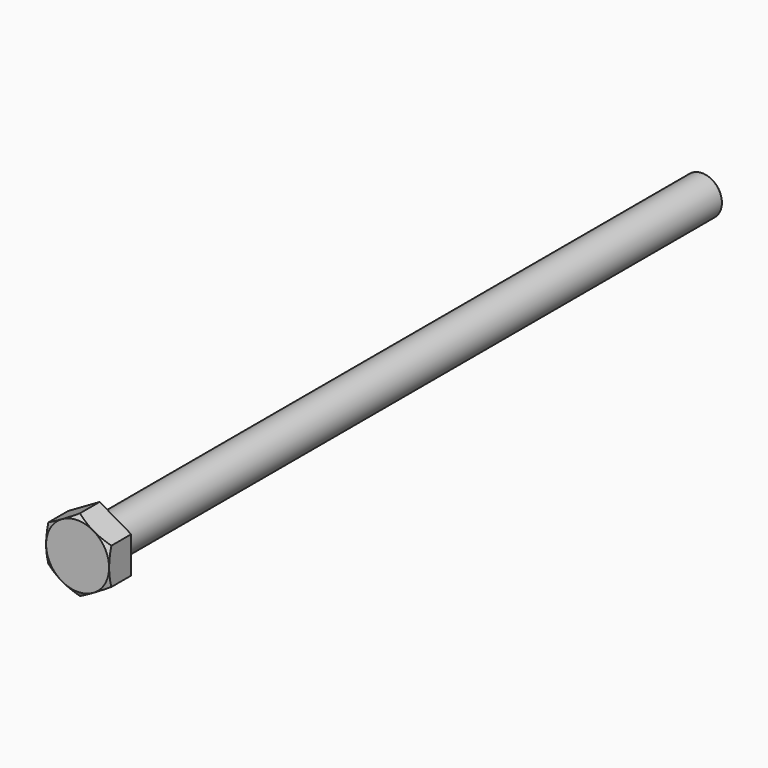
from build123d import *

# Parameters (mm, degrees)
F2_R     = 3.96875
F3_DEPTH = 152.4
F5_DEPTH = 5.55625
F6_SIZE  = 0.635


# Not quite as in the source:
# - a length typed as a fraction of an inch, garbled in the dataset ("3 / 203.2 mm" for 3/8 in), is restored


with BuildPart() as f3:
    # F2 (on Front) → F3 (new body)
    with BuildSketch(Plane.XZ):
        Circle(F2_R)
    extrude(amount=-F3_DEPTH)

    # F4 (on Front) → F5 (join)
    with BuildSketch(Plane.XZ):
        Polygon((0, -7.3323484187), (6.35, -3.6661742094), (6.35, 3.6661742094), (0, 7.3323484187), (-6.35, 3.6661742094), (-6.35, -3.6661742094), align=None)
    extrude(amount=F5_DEPTH)

    # F6
    f6_edges = [f3.edges().sort_by_distance(p)[0] for p in [
        (-3.96875, 152.4, 0),
    ]]
    chamfer(f6_edges, length=F6_SIZE)

    # F7 (on Top) → F8 (revolve, cut)
    with BuildSketch(Plane.XY):
        Polygon((13.4339599431, -5.55625), (13.4339599431, -1.4663238199), (6.35, -5.55625), align=None)
    revolve(axis=Axis((0, -2.778125, 0), (0, -1, 0)), mode=Mode.SUBTRACT)


solid = f3.part
